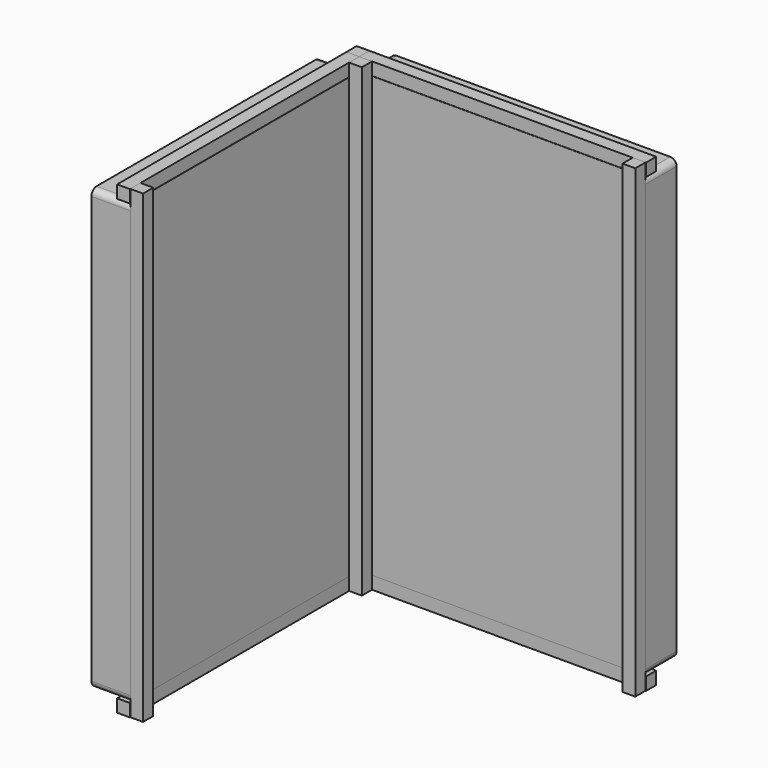
from build123d import *

# Parameters (mm, degrees)
F0_W      = 20
F0_H      = 20
F3_DEPTH  = 730
F4_DEPTH  = 730
F5_W      = 20
F5_H      = 20
F6_DEPTH  = 450
F8_DEPTH  = 61
F9_W      = 20
F9_H      = 20
F10_DEPTH = 730
F11_W     = 20
F11_H     = 20
F12_DEPTH = 450


# Not quite as in the source:
# - a feature of the source that left no trace in its solid (it failed there, or was rolled back) is left out
# - a pattern or mirror of a feature is missing from the dataset's text; its kind, count and spacing are read off the source's solid


with BuildPart() as f3:
    # F0 (on Top) → F3 (new body)
    with BuildSketch(Plane.XY):
        with Locations((-10, 10)):
            Rectangle(F0_W, F0_H)
    extrude(amount=F3_DEPTH)


with BuildPart() as f4:
    # F0 (on Top) → F4 (new body)
    with BuildSketch(Plane.XY):
        with Locations((10, -10)):
            Rectangle(F0_W, F0_H)
    extrude(amount=F4_DEPTH)


with BuildPart() as f4_copies_1:
    # F4_copies: instance of F4
    add(f4.part.mirror(Plane(origin=(0, -224.6, 0), x_dir=(0, 0, -1), z_dir=(0, -1, 0))))

    # F6_copies: F6 across plane


with BuildPart() as f6:
    # F5 (on face) → F6 (new body)
    with BuildSketch(Plane.YZ):
        with Locations((10, 10)):
            Rectangle(F5_W, F5_H)
    extrude(amount=F6_DEPTH)


with BuildPart() as f4_copies_1_1:
    add(f4_copies_1.part)
    add(f6.part.mirror(Plane(origin=(0, 0, 0), x_dir=(0.7071067812, -0.7071067812, 0), z_dir=(-0.7071067812, -0.7071067812, 0))))


with BuildPart() as f8:
    # F7 (on face) → F8 (new body)
    with BuildSketch(Plane(origin=(0, 0, 0), x_dir=(-1, 0, 0), z_dir=(0, 1, 0))):
        with BuildLine():
            Line((-439.2, 20), (-10, 20))
            ThreePointArc((-10, 20), (-2.9289321881, 22.9289321881), (0, 30))
            Line((0, 30), (0, 699.7))
            ThreePointArc((0, 699.7), (-2.9289321881, 706.7710678119), (-10, 709.7))
            Line((-10, 709.7), (-439.2, 709.7))
            ThreePointArc((-439.2, 709.7), (-446.2710678119, 706.7710678119), (-449.2, 699.7))
            Line((-449.2, 699.7), (-449.2, 30))
            ThreePointArc((-449.2, 30), (-446.2710678119, 22.9289321881), (-439.2, 20))
        make_face()
    extrude(amount=F8_DEPTH)


with BuildPart() as f8_copies_1:
    # F8_copies: instance of F8
    add(f8.part.mirror(Plane(origin=(0, 0, 0), x_dir=(-0.7071067812, 0.7071067812, 0), z_dir=(-0.7071067812, -0.7071067812, 0))))


with BuildPart() as f6_1:
    add(f6.part)

    # F9 (on Top) → F10 (join)
    with BuildSketch(Plane.XY):
        with Locations((439.2, -10)):
            Rectangle(F9_W, F9_H)
    extrude(amount=F10_DEPTH)


with BuildPart() as f12:
    # F11 (on face) → F12 (new body)
    with BuildSketch(Plane.YZ):
        with Locations((10, 720)):
            Rectangle(F11_W, F11_H)
    extrude(amount=F12_DEPTH)


with BuildPart() as f12_copies_1:
    # F12_copies: instance of F12
    add(f12.part.mirror(Plane(origin=(0, 0, 0), x_dir=(-0.7071067812, 0.7071067812, 0), z_dir=(-0.7071067812, -0.7071067812, 0))))


solid = Compound([f3.part, f4.part, f4_copies_1_1.part, f8.part, f8_copies_1.part, f6_1.part, f12.part, f12_copies_1.part])
